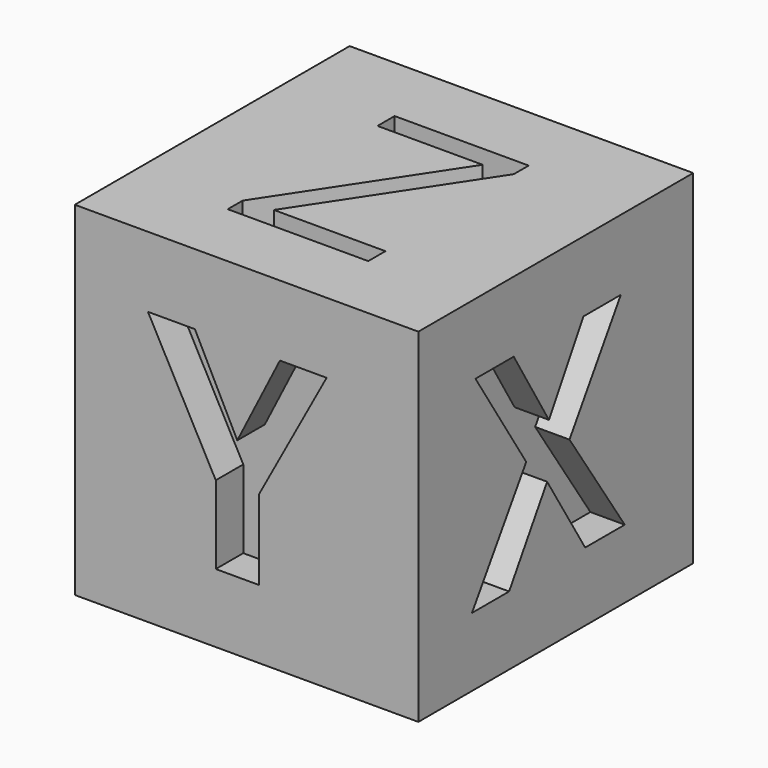
from build123d import *

# Parameters (mm, degrees)
F1_W          = 10
F1_H          = 10
F2_DEPTH      = 10
F4_TEXT_SIZE  = 8.3333333333
F5_DEPTH      = 1
F7_TEXT_SIZE  = 8.3333333333
F8_DEPTH      = 1
F10_TEXT_SIZE = 8.3333333333
F11_DEPTH     = 1


# Not quite as in the source:
# - Text() gives the source's letters only with a copy of the font that has no kerning and outlines rounded to 1/6400 em; it was checked with that copy


with BuildPart() as f2:
    # F1 (on Top) → F2 (new body)
    with BuildSketch(Plane.XY):
        Rectangle(F1_W, F1_H)
    extrude(amount=F2_DEPTH)

    # F4 (on offset) → F5 (cut)
    with BuildSketch(Plane.XZ.offset(5)):
        with Locations((-2.8704427083, 2)):
            Text('Y', F4_TEXT_SIZE, font='Open Sans', font_style=FontStyle.BOLD, text_align=(TextAlign.LEFT, TextAlign.BOTTOM))
    extrude(amount=-F5_DEPTH, mode=Mode.SUBTRACT)

    # F7 (on offset) → F8 (cut)
    with BuildSketch(Plane.YZ.offset(5)):
        with Locations((-3.0494791667, 2)):
            Text('X', F7_TEXT_SIZE, font='Open Sans', font_style=FontStyle.BOLD, text_align=(TextAlign.LEFT, TextAlign.BOTTOM))
    extrude(amount=-F8_DEPTH, mode=Mode.SUBTRACT)

    # F10 (on offset) → F11 (cut)
    with BuildSketch(Plane.XY.offset(10)):
        with Locations((-2.4817708333, -3)):
            Text('Z', F10_TEXT_SIZE, font='Open Sans', text_align=(TextAlign.LEFT, TextAlign.BOTTOM))
    extrude(amount=-F11_DEPTH, mode=Mode.SUBTRACT)


solid = f2.part
